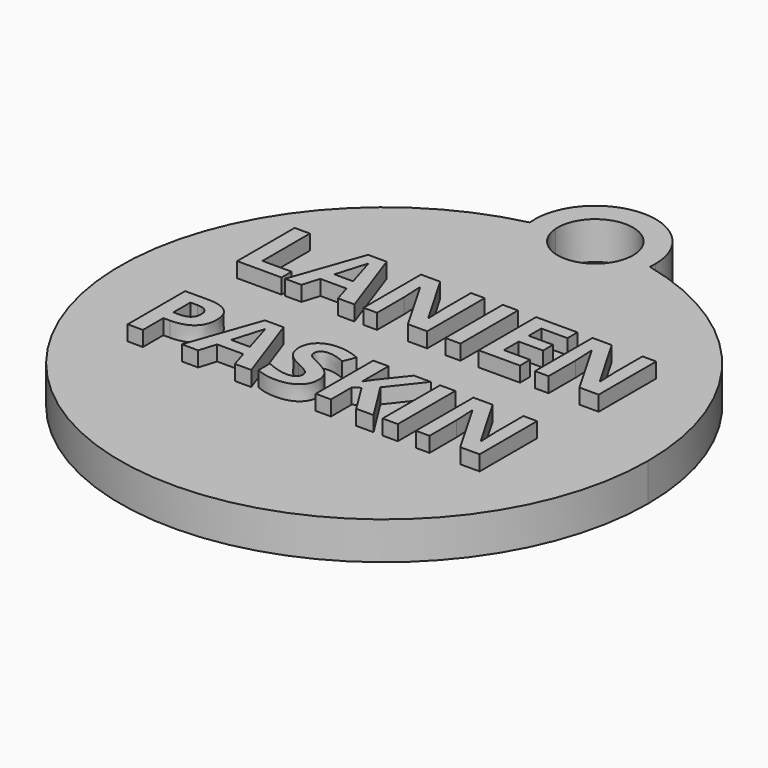
from build123d import *

# Parameters (mm, degrees)
F0_W         = 2.0203494433
F0_H         = 9.5262916476
F1_DEPTH     = 5
F0_TEXT_SIZE = 13.343897252
F2_DEPTH     = 7


# Not quite as in the source:
# - Text() gives the source's letters only with a copy of the font that has no kerning and outlines rounded to 1/6400 em; it was checked with that copy


with BuildPart() as f1:
    # F0 (on Top) → F1 (new body)
    with BuildSketch(Plane.XY):
        with BuildLine():
            ThreePointArc((-67.9475833832, 34.0857142857), (-81.7581545815, -27.415008831), (-25, 0))
            ThreePointArc((-25, 0), (-32.584991169, 21.7581545815), (-52.0524166168, 34.0857142857))
            ThreePointArc((-52.0524166168, 34.0857142857), (-60, 27), (-67.9475833832, 34.0857142857))
        make_face()
        with BuildLine():
            add(Edge.make_bspline(
                [(-78.1226804554, -3.9754388891), (-77.2209248989, -4.7218631417), (-77.2209248989, -6.2001167591)],
                knots=[0, 0, 0, 1, 1, 1], degree=2))
            add(Edge.make_bspline(
                [(-77.2209248989, -6.2001167591), (-77.2209248989, -7.738834911), (-78.1821024978, -8.5530211417)],
                knots=[0, 0, 0, 1, 1, 1], degree=2))
            add(Edge.make_bspline(
                [(-78.1821024978, -8.5530211417), (-79.1432800967, -9.3672073725), (-80.9155164505, -9.3672073725)],
                knots=[0, 0, 0, 1, 1, 1], degree=2))
            Line((-80.9155164505, -9.3672073725), (-81.780784788, -9.3672073725))
            Line((-81.780784788, -9.3672073725), (-81.780784788, -12.7553062841))
            Line((-81.780784788, -12.7553062841), (-83.8011342313, -12.7553062841))
            Line((-83.8011342313, -12.7553062841), (-83.8011342313, -3.2290146366))
            Line((-83.8011342313, -3.2290146366), (-80.7591426546, -3.2290146366))
            add(Edge.make_bspline(
                [(-80.7591426546, -3.2290146366), (-79.0244360118, -3.2290146366), (-78.1226804554, -3.9754388891)],
                knots=[0, 0, 0, 1, 1, 1], degree=2))
        make_face(mode=Mode.SUBTRACT)
        Polygon((-67.4131604187, -12.7553062841), (-69.5898836579, -12.7553062841), (-70.2800133439, -10.4868437513), (-73.7535965973, -10.4868437513), (-74.4437262833, -12.7553062841), (-76.6204495225, -12.7553062841), (-73.2573704182, -3.1893999416), (-70.7887494266, -3.1893999416), align=None, mode=Mode.SUBTRACT)
        with BuildLine():
            add(Edge.make_bspline(
                [(-61.0862766357, -8.5363412702), (-60.5910929486, -9.1774738335), (-60.5910929486, -10.1094616571)],
                knots=[0, 0, 0, 1, 1, 1], degree=2))
            add(Edge.make_bspline(
                [(-60.5910929486, -10.1094616571), (-60.5910929486, -11.4000667195), (-61.5199532964, -12.1433634961)],
                knots=[0, 0, 0, 1, 1, 1], degree=2))
            add(Edge.make_bspline(
                [(-61.5199532964, -12.1433634961), (-62.4488136441, -12.8866602727), (-64.102205913, -12.8866602727)],
                knots=[0, 0, 0, 1, 1, 1], degree=2))
            add(Edge.make_bspline(
                [(-64.102205913, -12.8866602727), (-65.6284141612, -12.8866602727), (-66.8001751387, -12.3112047037)],
                knots=[0, 0, 0, 1, 1, 1], degree=2))
            Line((-66.8001751387, -12.3112047037), (-66.8001751387, -10.4347191527))
            add(Edge.make_bspline(
                [(-66.8001751387, -10.4347191527), (-65.8369125558, -10.8663108294), (-65.1686752012, -11.0414494808)],
                knots=[0, 0, 0, 1, 1, 1], degree=2))
            add(Edge.make_bspline(
                [(-65.1686752012, -11.0414494808), (-64.5004378466, -11.2165881323), (-63.9458321171, -11.2165881323)],
                knots=[0, 0, 0, 1, 1, 1], degree=2))
            add(Edge.make_bspline(
                [(-63.9458321171, -11.2165881323), (-63.2828072224, -11.2165881323), (-62.9273174597, -10.9632625829)],
                knots=[0, 0, 0, 1, 1, 1], degree=2))
            add(Edge.make_bspline(
                [(-62.9273174597, -10.9632625829), (-62.5718276969, -10.7099370335), (-62.5718276969, -10.2074559026)],
                knots=[0, 0, 0, 1, 1, 1], degree=2))
            add(Edge.make_bspline(
                [(-62.5718276969, -10.2074559026), (-62.5718276969, -9.9280680539), (-62.7282014928, -9.7091447396)],
                knots=[0, 0, 0, 1, 1, 1], degree=2))
            add(Edge.make_bspline(
                [(-62.7282014928, -9.7091447396), (-62.8845752888, -9.4902214253), (-63.1879404529, -9.2890204745)],
                knots=[0, 0, 0, 1, 1, 1], degree=2))
            add(Edge.make_bspline(
                [(-63.1879404529, -9.2890204745), (-63.4913056169, -9.0878195238), (-64.4232934406, -8.6437179434)],
                knots=[0, 0, 0, 1, 1, 1], degree=2))
            add(Edge.make_bspline(
                [(-64.4232934406, -8.6437179434), (-65.2948167299, -8.2329761061), (-65.7316208665, -7.8555940119)],
                knots=[0, 0, 0, 1, 1, 1], degree=2))
            add(Edge.make_bspline(
                [(-65.7316208665, -7.8555940119), (-66.1684250031, -7.4782119178), (-66.4290479963, -6.9757307869)],
                knots=[0, 0, 0, 1, 1, 1], degree=2))
            add(Edge.make_bspline(
                [(-66.4290479963, -6.9757307869), (-66.6896709895, -6.473249656), (-66.6896709895, -5.8039698094)],
                knots=[0, 0, 0, 1, 1, 1], degree=2))
            add(Edge.make_bspline(
                [(-66.6896709895, -5.8039698094), (-66.6896709895, -4.5383845544), (-65.8327425879, -3.8159376173)],
                knots=[0, 0, 0, 1, 1, 1], degree=2))
            add(Edge.make_bspline(
                [(-65.8327425879, -3.8159376173), (-64.9758141862, -3.0934906801), (-63.4642008257, -3.0934906801)],
                knots=[0, 0, 0, 1, 1, 1], degree=2))
            add(Edge.make_bspline(
                [(-63.4642008257, -3.0934906801), (-62.721946541, -3.0934906801), (-62.0474542346, -3.2686293316)],
                knots=[0, 0, 0, 1, 1, 1], degree=2))
            add(Edge.make_bspline(
                [(-62.0474542346, -3.2686293316), (-61.3729619282, -3.443767983), (-60.6369625954, -3.7627705267)],
                knots=[0, 0, 0, 1, 1, 1], degree=2))
            Line((-60.6369625954, -3.7627705267), (-61.2874775864, -5.3348484217))
            add(Edge.make_bspline(
                [(-61.2874775864, -5.3348484217), (-62.0505817105, -5.0221008298), (-62.5488928735, -4.8980442851)],
                knots=[0, 0, 0, 1, 1, 1], degree=2))
            add(Edge.make_bspline(
                [(-62.5488928735, -4.8980442851), (-63.0472040365, -4.7739877403), (-63.528835328, -4.7739877403)],
                knots=[0, 0, 0, 1, 1, 1], degree=2))
            add(Edge.make_bspline(
                [(-63.528835328, -4.7739877403), (-64.102205913, -4.7739877403), (-64.408698553, -5.0408656853)],
                knots=[0, 0, 0, 1, 1, 1], degree=2))
            add(Edge.make_bspline(
                [(-64.408698553, -5.0408656853), (-64.715191193, -5.3077436304), (-64.715191193, -5.7372503232)],
                knots=[0, 0, 0, 1, 1, 1], degree=2))
            add(Edge.make_bspline(
                [(-64.715191193, -5.7372503232), (-64.715191193, -6.0041282682), (-64.5911346483, -6.203244235)],
                knots=[0, 0, 0, 1, 1, 1], degree=2))
            add(Edge.make_bspline(
                [(-64.5911346483, -6.203244235), (-64.4670781035, -6.4023602018), (-64.1970726825, -6.587923773)],
                knots=[0, 0, 0, 1, 1, 1], degree=2))
            add(Edge.make_bspline(
                [(-64.1970726825, -6.587923773), (-63.9270672616, -6.7734873441), (-62.9179350319, -7.2551186356)],
                knots=[0, 0, 0, 1, 1, 1], degree=2))
            add(Edge.make_bspline(
                [(-62.9179350319, -7.2551186356), (-61.5814603228, -7.8952087069), (-61.0862766357, -8.5363412702)],
                knots=[0, 0, 0, 1, 1, 1], degree=2))
        make_face(mode=Mode.SUBTRACT)
        Polygon((-54.5508944581, -7.4448521746), (-51.2024102414, -12.7553062841), (-53.4958925816, -12.7553062841), (-55.9916183645, -8.7417121888), (-56.8443767983, -9.3546974688), (-56.8443767983, -12.7553062841), (-58.8647262416, -12.7553062841), (-58.8647262416, -3.2290146366), (-56.8443767983, -3.2290146366), (-56.8443767983, -7.5887160669), (-56.049997915, -6.4669947041), (-53.4687877903, -3.2290146366), (-51.2274300488, -3.2290146366), align=None, mode=Mode.SUBTRACT)
        with Locations((-48.9933697511, -7.9921604604)):
            Rectangle(F0_W, F0_H, mode=Mode.SUBTRACT)
        with BuildLine():
            Line((-37.1350235603, -3.2290146366), (-37.1350235603, -12.7553062841))
            Line((-37.1350235603, -12.7553062841), (-39.7016387974, -12.7553062841))
            Line((-39.7016387974, -12.7553062841), (-43.8465868813, -5.5496017681))
            Line((-43.8465868813, -5.5496017681), (-43.9049664318, -5.5496017681))
            add(Edge.make_bspline(
                [(-43.9049664318, -5.5496017681), (-43.779867395, -7.4573620783), (-43.779867395, -8.2725908011)],
                knots=[0, 0, 0, 1, 1, 1], degree=2))
            Line((-43.779867395, -8.2725908011), (-43.779867395, -12.7553062841))
            Line((-43.779867395, -12.7553062841), (-45.5854634919, -12.7553062841))
            Line((-45.5854634919, -12.7553062841), (-45.5854634919, -3.2290146366))
            Line((-45.5854634919, -3.2290146366), (-43.0376131104, -3.2290146366))
            Line((-43.0376131104, -3.2290146366), (-38.9010049623, -10.3638296985))
            Line((-38.9010049623, -10.3638296985), (-38.8551353155, -10.3638296985))
            add(Edge.make_bspline(
                [(-38.8551353155, -10.3638296985), (-38.9531295609, -8.506109003), (-38.9531295609, -7.738834911)],
                knots=[0, 0, 0, 1, 1, 1], degree=2))
            Line((-38.9531295609, -7.738834911), (-38.9531295609, -3.2290146366))
            Line((-38.9531295609, -3.2290146366), (-37.1350235603, -3.2290146366))
        make_face(mode=Mode.SUBTRACT)
        Polygon((-77.9173095367, 5.3923939786), (-83.8011342313, 5.3923939786), (-83.8011342313, 14.9186856261), (-81.780784788, 14.9186856261), (-81.780784788, 7.0603811351), (-77.9173095367, 7.0603811351), align=None, mode=Mode.SUBTRACT)
        Polygon((-68.2534089488, 5.3923939786), (-70.430132188, 5.3923939786), (-71.120261874, 7.6608565114), (-74.5938451274, 7.6608565114), (-75.2839748134, 5.3923939786), (-77.4606980526, 5.3923939786), (-74.0976189483, 14.9583003211), (-71.6289979567, 14.9583003211), align=None, mode=Mode.SUBTRACT)
        with BuildLine():
            Line((-58.6041032484, 14.9186856261), (-58.6041032484, 5.3923939786))
            Line((-58.6041032484, 5.3923939786), (-61.1707184855, 5.3923939786))
            Line((-61.1707184855, 5.3923939786), (-65.3156665694, 12.5980984946))
            Line((-65.3156665694, 12.5980984946), (-65.3740461198, 12.5980984946))
            add(Edge.make_bspline(
                [(-65.3740461198, 12.5980984946), (-65.2489470831, 10.6903381844), (-65.2489470831, 9.8751094617)],
                knots=[0, 0, 0, 1, 1, 1], degree=2))
            Line((-65.2489470831, 9.8751094617), (-65.2489470831, 5.3923939786))
            Line((-65.2489470831, 5.3923939786), (-67.05454318, 5.3923939786))
            Line((-67.05454318, 5.3923939786), (-67.05454318, 14.9186856261))
            Line((-67.05454318, 14.9186856261), (-64.5066927985, 14.9186856261))
            Line((-64.5066927985, 14.9186856261), (-60.3700846503, 7.7838705642))
            Line((-60.3700846503, 7.7838705642), (-60.3242150035, 7.7838705642))
            add(Edge.make_bspline(
                [(-60.3242150035, 7.7838705642), (-60.422209249, 9.6415912597), (-60.422209249, 10.4088653517)],
                knots=[0, 0, 0, 1, 1, 1], degree=2))
            Line((-60.422209249, 10.4088653517), (-60.422209249, 14.9186856261))
            Line((-60.422209249, 14.9186856261), (-58.6041032484, 14.9186856261))
        make_face(mode=Mode.SUBTRACT)
        with Locations((-55.1961969893, 10.1555398023)):
            Rectangle(F0_W, F0_H, mode=Mode.SUBTRACT)
        Polygon((-46.3026979692, 7.0603811351), (-46.3026979692, 5.3923939786), (-51.7882907302, 5.3923939786), (-51.7882907302, 14.9186856261), (-46.3026979692, 14.9186856261), (-46.3026979692, 13.2632083733), (-49.7679412869, 13.2632083733), (-49.7679412869, 11.1719694758), (-46.542471123, 11.1719694758), (-46.542471123, 9.516492223), (-49.7679412869, 9.516492223), (-49.7679412869, 7.0603811351), align=None, mode=Mode.SUBTRACT)
        with BuildLine():
            Line((-35.8652683374, 14.9186856261), (-35.8652683374, 5.3923939786))
            Line((-35.8652683374, 5.3923939786), (-38.4318835745, 5.3923939786))
            Line((-38.4318835745, 5.3923939786), (-42.5768316584, 12.5980984946))
            Line((-42.5768316584, 12.5980984946), (-42.6352112089, 12.5980984946))
            add(Edge.make_bspline(
                [(-42.6352112089, 12.5980984946), (-42.5101121721, 10.6903381844), (-42.5101121721, 9.8751094617)],
                knots=[0, 0, 0, 1, 1, 1], degree=2))
            Line((-42.5101121721, 9.8751094617), (-42.5101121721, 5.3923939786))
            Line((-42.5101121721, 5.3923939786), (-44.315708269, 5.3923939786))
            Line((-44.315708269, 5.3923939786), (-44.315708269, 14.9186856261))
            Line((-44.315708269, 14.9186856261), (-41.7678578875, 14.9186856261))
            Line((-41.7678578875, 14.9186856261), (-37.6312497394, 7.7838705642))
            Line((-37.6312497394, 7.7838705642), (-37.5853800926, 7.7838705642))
            add(Edge.make_bspline(
                [(-37.5853800926, 7.7838705642), (-37.683374338, 9.6415912597), (-37.683374338, 10.4088653517)],
                knots=[0, 0, 0, 1, 1, 1], degree=2))
            Line((-37.683374338, 10.4088653517), (-37.683374338, 14.9186856261))
            Line((-37.683374338, 14.9186856261), (-35.8652683374, 14.9186856261))
        make_face(mode=Mode.SUBTRACT)
        with BuildLine():
            ThreePointArc((-67.9475833832, 34.0857142857), (-60, 27), (-52.0524166168, 34.0857142857))
            ThreePointArc((-52.0524166168, 34.0857142857), (-53.5265973231, 34.3961488801), (-55.0127714129, 34.6428571429))
            ThreePointArc((-55.0127714129, 34.6428571429), (-60, 30), (-64.9872285871, 34.6428571429))
            ThreePointArc((-64.9872285871, 34.6428571429), (-66.4734026769, 34.3961488801), (-67.9475833832, 34.0857142857))
        make_face()
        with BuildLine():
            ThreePointArc((-55.0127714129, 34.6428571429), (-53.5265973231, 34.3961488801), (-52.0524166168, 34.0857142857))
            ThreePointArc((-52.0524166168, 34.0857142857), (-52.0131149042, 34.5421064892), (-52, 35))
            ThreePointArc((-52, 35), (-60.4578935108, 42.9868850958), (-67.9475833832, 34.0857142857))
            ThreePointArc((-67.9475833832, 34.0857142857), (-66.4734026769, 34.3961488801), (-64.9872285871, 34.6428571429))
            ThreePointArc((-64.9872285871, 34.6428571429), (-60.1786855684, 39.9968061267), (-55, 35))
            ThreePointArc((-55, 35), (-55.0031938733, 34.8213144316), (-55.0127714129, 34.6428571429))
        make_face()
    extrude(amount=F1_DEPTH)



with BuildPart() as f1b:
    # F0 (on Top) → F1, piece 2 (new body)
    with BuildSketch(Plane.XY):
        with BuildLine():
            Line((-74.0851090447, 9.3538634753), (-71.6039781494, 9.3538634753))
            add(Edge.make_bspline(
                [(-71.6039781494, 9.3538634753), (-72.5609857804, 12.4354697469), (-72.6819148493, 12.8399566323)],
                knots=[0, 0, 0, 1, 1, 1], degree=2))
            add(Edge.make_bspline(
                [(-72.6819148493, 12.8399566323), (-72.8028439181, 13.2444435178), (-72.8549685167, 13.4779617197)],
                knots=[0, 0, 0, 1, 1, 1], degree=2))
            add(Edge.make_bspline(
                [(-72.8549685167, 13.4779617197), (-73.0697218631, 12.6439681414), (-74.0851090447, 9.3538634753)],
                knots=[0, 0, 0, 1, 1, 1], degree=2))
        make_face()
    extrude(amount=F1_DEPTH)


with BuildPart() as f1c:
    # F0 (on Top) → F1, piece 3 (new body)
    with BuildSketch(Plane.XY):
        with BuildLine():
            Line((-73.2448605146, -8.7938367875), (-70.7637296193, -8.7938367875))
            add(Edge.make_bspline(
                [(-70.7637296193, -8.7938367875), (-71.7207372503, -5.7122305158), (-71.8416663192, -5.3077436304)],
                knots=[0, 0, 0, 1, 1, 1], degree=2))
            add(Edge.make_bspline(
                [(-71.8416663192, -5.3077436304), (-71.962595388, -4.9032567449), (-72.0147199867, -4.669738543)],
                knots=[0, 0, 0, 1, 1, 1], degree=2))
            add(Edge.make_bspline(
                [(-72.0147199867, -4.669738543), (-72.2294733331, -5.5037321213), (-73.2448605146, -8.7938367875)],
                knots=[0, 0, 0, 1, 1, 1], degree=2))
        make_face()
    extrude(amount=F1_DEPTH)


with BuildPart() as f1d:
    # F0 (on Top) → F1, piece 4 (new body)
    with BuildSketch(Plane.XY):
        with BuildLine():
            Line((-81.780784788, -4.8844918894), (-81.780784788, -7.7117301197))
            Line((-81.780784788, -7.7117301197), (-81.1156749093, -7.7117301197))
            add(Edge.make_bspline(
                [(-81.1156749093, -7.7117301197), (-80.1857720696, -7.7117301197), (-79.7229056336, -7.3437304533)],
                knots=[0, 0, 0, 1, 1, 1], degree=2))
            add(Edge.make_bspline(
                [(-79.7229056336, -7.3437304533), (-79.2600391977, -6.9757307869), (-79.2600391977, -6.2730911972)],
                knots=[0, 0, 0, 1, 1, 1], degree=2))
            add(Edge.make_bspline(
                [(-79.2600391977, -6.2730911972), (-79.2600391977, -5.5621116717), (-79.6478462116, -5.2233017806)],
                knots=[0, 0, 0, 1, 1, 1], degree=2))
            add(Edge.make_bspline(
                [(-79.6478462116, -5.2233017806), (-80.0356532255, -4.8844918894), (-80.8633918519, -4.8844918894)],
                knots=[0, 0, 0, 1, 1, 1], degree=2))
            Line((-80.8633918519, -4.8844918894), (-81.780784788, -4.8844918894))
        make_face()
    extrude(amount=F1_DEPTH)


with BuildPart() as f1_1:
    add(f1.part)

    add(f1b.part)  # F2 merges F1b

    add(f1c.part)  # F2 merges F1c

    add(f1d.part)  # F2 merges F1d
    # F0 (on Top) → F2 (join)
    with BuildSketch(Plane.XY):
        with Locations((-85, -12.7553062841)):
            Text('PASKIN', F0_TEXT_SIZE, font='Open Sans', font_style=FontStyle.BOLD, text_align=(TextAlign.LEFT, TextAlign.BOTTOM))
        with Locations((-85, 5.3923939786)):
            Text('LANIEN', F0_TEXT_SIZE, font='Open Sans', font_style=FontStyle.BOLD, text_align=(TextAlign.LEFT, TextAlign.BOTTOM))
    extrude(amount=F2_DEPTH)


solid = f1_1.part
